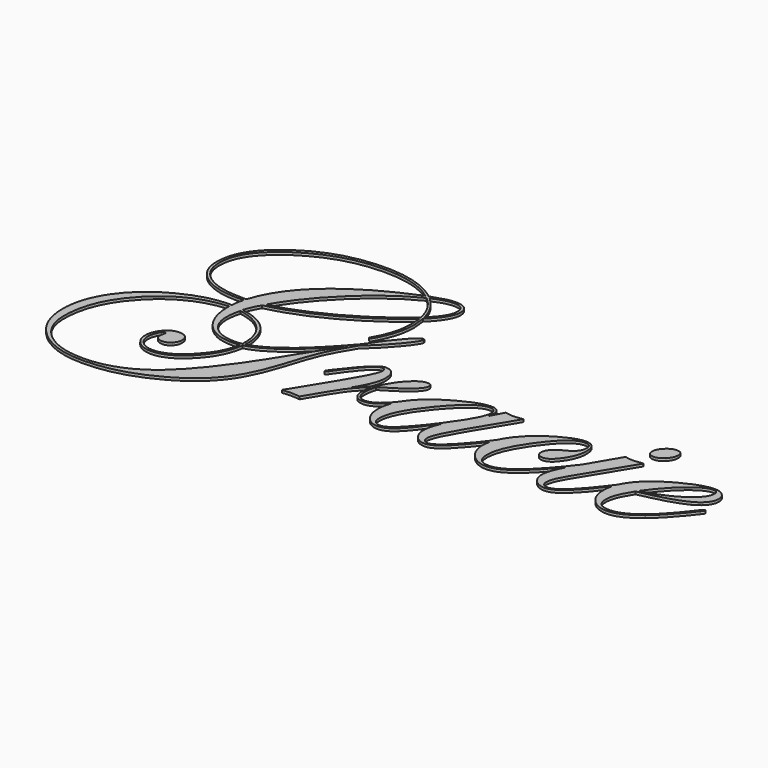
from build123d import *

# Parameters (mm, degrees)
F1_DEPTH = 1.5


# Not quite as in the source:
# - ends of sketch curves that miss each other by under 0.0002 mm in the source are joined


with BuildPart() as f1:
    # F0 (on Top) → F1 (new body)
    with BuildSketch(Plane.XY):
        with BuildLine():
            add(Edge.make_bspline(
                [(-28.4636718, 33.839658), (-28.4636718, 32.4505066), (-30.630749, 29.1998908), (-34.964878, 24.087836)],
                knots=[0, 0, 0, 0, 1, 1, 1, 1], degree=3))
            add(Edge.make_bspline(
                [(-29.1304218, 34.3397078), (-28.7970468, 34.3397078), (-28.5747714, 34.173033), (-28.4636718, 33.839658)],
                knots=[0, 0, 0, 0, 1, 1, 1, 1], degree=3))
            add(Edge.make_bspline(
                [(-36.8818668, 27.8385016), (-33.1033882, 32.172656), (-30.5195732, 34.3397078), (-29.1304218, 34.3397078)],
                knots=[0, 0, 0, 0, 1, 1, 1, 1], degree=3))
            add(Edge.make_bspline(
                [(-47.967265, 12.8356868), (-44.3554866, 18.5034174), (-40.6603454, 23.5043472), (-36.8818668, 27.8385016)],
                knots=[0, 0, 0, 0, 1, 1, 1, 1], degree=3))
            add(Edge.make_bspline(
                [(-88.7248924, -20.0871328), (-77.6672818, -17.0865546), (-64.081406, -6.1122814), (-47.967265, 12.8356868)],
                knots=[0, 0, 0, 0, 1, 1, 1, 1], degree=3))
            Line((-88.7248924, -20.0871328), (-88.7248924, -18.4201562))
            add(Edge.make_bspline(
                [(-110.729014, 5.5009796), (-96.0595996, 3.0005274), (-88.7248924, -4.973193), (-88.7248924, -18.4201562)],
                knots=[0, 0, 0, 0, 1, 1, 1, 1], degree=3))
            add(Edge.make_bspline(
                [(-106.6449226, 14.5026634), (-108.4230242, 11.6132356), (-109.784388, 8.6126828), (-110.729014, 5.5009796)],
                knots=[0, 0, 0, 0, 1, 1, 1, 1], degree=3))
            add(Edge.make_bspline(
                [(-74.055478, 27.0883634), (-85.4465144, 21.0316826), (-96.3096372, 16.8364408), (-106.6449226, 14.5026634)],
                knots=[0, 0, 0, 0, 1, 1, 1, 1], degree=3))
            add(Edge.make_bspline(
                [(-42.9663352, 48.5090216), (-52.2458442, 40.3408388), (-62.6088918, 33.2006194), (-74.055478, 27.0883634)],
                knots=[0, 0, 0, 0, 1, 1, 1, 1], degree=3))
            add(Edge.make_bspline(
                [(-42.6329348, 42.1745156), (-42.6329348, 44.4527178), (-42.7440852, 46.5642198), (-42.9663352, 48.5090216)],
                knots=[0, 0, 0, 0, 1, 1, 1, 1], degree=3))
            add(Edge.make_bspline(
                [(-48.800766, 20.8371948), (-44.688887, 27.6162262), (-42.6329348, 34.7286834), (-42.6329348, 42.1745156)],
                knots=[0, 0, 0, 0, 1, 1, 1, 1], degree=3))
            add(Edge.make_bspline(
                [(-49.1341664, 20.0036938), (-49.0786166, 20.281519), (-48.9674662, 20.5593442), (-48.800766, 20.8371948)],
                knots=[0, 0, 0, 0, 1, 1, 1, 1], degree=3))
            add(Edge.make_bspline(
                [(-48.6340912, 19.503644), (-48.9119164, 19.503644), (-49.0786166, 19.6703188), (-49.1341664, 20.0036938)],
                knots=[0, 0, 0, 0, 1, 1, 1, 1], degree=3))
            add(Edge.make_bspline(
                [(-46.3836766, 22.5875596), (-47.4394276, 20.5316074), (-48.1895658, 19.503644), (-48.6340912, 19.503644)],
                knots=[0, 0, 0, 0, 1, 1, 1, 1], degree=3))
            add(Edge.make_bspline(
                [(-41.1326838, 41.8411406), (-41.1326838, 35.840035), (-42.8830232, 29.4221662), (-46.3836766, 22.5875596)],
                knots=[0, 0, 0, 0, 1, 1, 1, 1], degree=3))
            add(Edge.make_bspline(
                [(-41.7994846, 49.5092482), (-41.3549592, 46.4531202), (-41.1326838, 43.8970928), (-41.1326838, 41.8411406)],
                knots=[0, 0, 0, 0, 1, 1, 1, 1], degree=3))
            add(Edge.make_bspline(
                [(-32.381063, 64.845438), (-32.381063, 60.733559), (-35.5205538, 55.6215042), (-41.7994846, 49.5092482)],
                knots=[0, 0, 0, 0, 1, 1, 1, 1], degree=3))
            add(Edge.make_bspline(
                [(-40.4659084, 71.5133698), (-35.076003, 71.5133698), (-32.381063, 69.2907174), (-32.381063, 64.845438)],
                knots=[0, 0, 0, 0, 1, 1, 1, 1], degree=3))
            add(Edge.make_bspline(
                [(-53.3850088, 68.262754), (-47.550578, 70.4298312), (-43.2442112, 71.5133698), (-40.4659084, 71.5133698)],
                knots=[0, 0, 0, 0, 1, 1, 1, 1], degree=3))
            add(Edge.make_bspline(
                [(-85.8077278, 78.1812762), (-72.5830146, 78.1812762), (-61.7754416, 74.8751106), (-53.3850088, 68.262754)],
                knots=[0, 0, 0, 0, 1, 1, 1, 1], degree=3))
            add(Edge.make_bspline(
                [(-130.0660086, 65.0121382), (-117.230271, 73.791572), (-102.4774938, 78.1812762), (-85.8077278, 78.1812762)],
                knots=[0, 0, 0, 0, 1, 1, 1, 1], degree=3))
            add(Edge.make_bspline(
                [(-149.3195896, 34.8398338), (-149.3195896, 46.175295), (-142.9017208, 56.2327298), (-130.0660086, 65.0121382)],
                knots=[0, 0, 0, 0, 1, 1, 1, 1], degree=3))
            add(Edge.make_bspline(
                [(-141.4014444, 19.0868808), (-146.6802248, 23.032085), (-149.3195896, 28.2830524), (-149.3195896, 34.8398338)],
                knots=[0, 0, 0, 0, 1, 1, 1, 1], degree=3))
            add(Edge.make_bspline(
                [(-119.9807862, 13.1691126), (-128.9268948, 13.1691126), (-136.0671142, 15.141702), (-141.4014444, 19.0868808)],
                knots=[0, 0, 0, 0, 1, 1, 1, 1], degree=3))
            add(Edge.make_bspline(
                [(-116.39677, 13.3357874), (-117.3969712, 13.2246878), (-118.5916348, 13.1691126), (-119.9807862, 13.1691126)],
                knots=[0, 0, 0, 0, 1, 1, 1, 1], degree=3))
            add(Edge.make_bspline(
                [(-117.563646, 6.0010802), (-117.5636714, 7.3902316), (-117.1746958, 9.835134), (-116.39677, 13.3357874)],
                knots=[0, 0, 0, 0, 1, 1, 1, 1], degree=3))
            add(Edge.make_bspline(
                [(-119.3139854, 6.1678312), (-118.6471846, 6.1678312), (-118.0637466, 6.1122306), (-117.563646, 6.0010802)],
                knots=[0, 0, 0, 0, 1, 1, 1, 1], degree=3))
            add(Edge.make_bspline(
                [(-145.068798, -1.0002012), (-135.789289, 3.7784786), (-127.204343, 6.1678312), (-119.3139854, 6.1678312)],
                knots=[0, 0, 0, 0, 1, 1, 1, 1], degree=3))
            add(Edge.make_bspline(
                [(-166.9062194, -19.8370444), (-161.5718892, -12.0578118), (-154.2927572, -5.7788556), (-145.068798, -1.0002012)],
                knots=[0, 0, 0, 0, 1, 1, 1, 1], degree=3))
            add(Edge.make_bspline(
                [(-174.907702, -44.3416436), (-174.907702, -35.72891), (-172.2405496, -27.5607018), (-166.9062194, -19.8370444)],
                knots=[0, 0, 0, 0, 1, 1, 1, 1], degree=3))
            add(Edge.make_bspline(
                [(-164.3224044, -68.8462428), (-171.3792864, -62.622811), (-174.907702, -54.4546282), (-174.907702, -44.3416436)],
                knots=[0, 0, 0, 0, 1, 1, 1, 1], degree=3))
            add(Edge.make_bspline(
                [(-136.5672148, -78.1813016), (-148.013801, -78.1813016), (-157.2655224, -75.0696238), (-164.3224044, -68.8462428)],
                knots=[0, 0, 0, 0, 1, 1, 1, 1], degree=3))
            add(Edge.make_bspline(
                [(-96.9764634, -67.4293038), (-109.8677762, -74.5973108), (-123.0646764, -78.1813016), (-136.5672148, -78.1813016)],
                knots=[0, 0, 0, 0, 1, 1, 1, 1], degree=3))
            add(Edge.make_bspline(
                [(-76.0559058, -50.3427746), (-81.0012604, -56.7328304), (-87.974805, -62.4283232), (-96.9764634, -67.4293038)],
                knots=[0, 0, 0, 0, 1, 1, 1, 1], degree=3))
            add(Edge.make_bspline(
                [(-63.4702058, -24.4212364), (-66.8597342, -35.3121722), (-71.054976, -43.9526934), (-76.0559058, -50.3427746)],
                knots=[0, 0, 0, 0, 1, 1, 1, 1], degree=3))
            add(Edge.make_bspline(
                [(-56.6355992, -4.834255), (-58.469276, -8.9461086), (-60.7474782, -15.4751278), (-63.4702058, -24.4212364)],
                knots=[0, 0, 0, 0, 1, 1, 1, 1], degree=3))
            add(Edge.make_bspline(
                [(-47.9673158, 10.918698), (-51.9124946, 4.584192), (-54.8019224, -0.6668008), (-56.6355992, -4.834255)],
                knots=[0, 0, 0, 0, 1, 1, 1, 1], degree=3))
            add(Edge.make_bspline(
                [(-34.964878, 24.087836), (-39.2434572, 19.031331), (-43.5776116, 14.6416268), (-47.9673158, 10.918698)],
                knots=[0, 0, 0, 0, 1, 1, 1, 1], degree=3))
        make_face()
        with BuildLine():
            add(Edge.make_bspline(
                [(-50.8845312, 7.5014074), (-65.8317708, -9.1128088), (-78.556358, -18.8368432), (-89.0583436, -21.6707212)],
                knots=[0, 0, 0, 0, 1, 1, 1, 1], degree=3))
            add(Edge.make_bspline(
                [(-64.6371072, -13.1691634), (-60.3029528, -5.8344562), (-55.7187608, 1.0557256), (-50.8845312, 7.5014074)],
                knots=[0, 0, 0, 0, 1, 1, 1, 1], degree=3))
            add(Edge.make_bspline(
                [(-101.9774186, -62.5117368), (-91.253183, -53.2322278), (-78.806421, -36.7847118), (-64.6371072, -13.1691634)],
                knots=[0, 0, 0, 0, 1, 1, 1, 1], degree=3))
            add(Edge.make_bspline(
                [(-137.7340908, -76.4309876), (-124.620528, -76.4309876), (-112.7016288, -71.7912458), (-101.9774186, -62.5117368)],
                knots=[0, 0, 0, 0, 1, 1, 1, 1], degree=3))
            add(Edge.make_bspline(
                [(-161.2384888, -68.9296056), (-155.2373578, -73.9305354), (-147.4025754, -76.4309876), (-137.7340908, -76.4309876)],
                knots=[0, 0, 0, 0, 1, 1, 1, 1], degree=3))
            add(Edge.make_bspline(
                [(-170.1568352, -49.3425988), (-170.1568352, -57.399682), (-167.1840446, -63.9286758), (-161.2384888, -68.9296056)],
                knots=[0, 0, 0, 0, 1, 1, 1, 1], degree=3))
            add(Edge.make_bspline(
                [(-154.4872196, -13.0858006), (-164.93363, -23.8100362), (-170.1568352, -35.8956356), (-170.1568352, -49.3425988)],
                knots=[0, 0, 0, 0, 1, 1, 1, 1], degree=3))
            add(Edge.make_bspline(
                [(-117.7303462, 4.4174664), (-131.7329852, 3.5284156), (-143.9852594, -2.3060152), (-154.4872196, -13.0858006)],
                knots=[0, 0, 0, 0, 1, 1, 1, 1], degree=3))
            add(Edge.make_bspline(
                [(-111.5625404, -15.1695404), (-115.6744194, -10.3352854), (-117.7303462, -3.8062916), (-117.7303462, 4.4174664)],
                knots=[0, 0, 0, 0, 1, 1, 1, 1], degree=3))
            add(Edge.make_bspline(
                [(-94.7260488, -22.3375474), (-101.838506, -22.3375474), (-107.4506614, -19.9481948), (-111.5625404, -15.1695404)],
                knots=[0, 0, 0, 0, 1, 1, 1, 1], degree=3))
            add(Edge.make_bspline(
                [(-90.4752572, -22.004147), (-91.6977084, -22.226397), (-93.1146474, -22.3375474), (-94.7260488, -22.3375474)],
                knots=[0, 0, 0, 0, 1, 1, 1, 1], degree=3))
            add(Edge.make_bspline(
                [(-100.643817, -41.2577534), (-94.6427114, -35.0899222), (-91.253183, -28.6720534), (-90.4752572, -22.004147)],
                knots=[0, 0, 0, 0, 1, 1, 1, 1], degree=3))
            add(Edge.make_bspline(
                [(-118.0637466, -50.5094748), (-112.396016, -50.5094748), (-106.5893728, -47.4255592), (-100.643817, -41.2577534)],
                knots=[0, 0, 0, 0, 1, 1, 1, 1], degree=3))
            add(Edge.make_bspline(
                [(-125.1484162, -47.9256852), (-123.2591642, -49.6482116), (-120.8976246, -50.5094748), (-118.0637466, -50.5094748)],
                knots=[0, 0, 0, 0, 1, 1, 1, 1], degree=3))
            add(Edge.make_bspline(
                [(-127.9822688, -41.4244028), (-127.9822688, -44.0360054), (-127.0376428, -46.203108), (-125.1484162, -47.9256852)],
                knots=[0, 0, 0, 0, 1, 1, 1, 1], degree=3))
            add(Edge.make_bspline(
                [(-126.73203, -36.3401356), (-127.565531, -38.118288), (-127.9822688, -39.8130268), (-127.9822688, -41.4244028)],
                knots=[0, 0, 0, 0, 1, 1, 1, 1], degree=3))
            add(Edge.make_bspline(
                [(-124.2315778, -33.5896458), (-125.0650534, -33.5896458), (-125.8985544, -34.5064842), (-126.73203, -36.3401356)],
                knots=[0, 0, 0, 0, 1, 1, 1, 1], degree=3))
            add(Edge.make_bspline(
                [(-123.7315026, -34.0896956), (-123.7315026, -33.7563206), (-123.8982028, -33.5896458), (-124.2315778, -33.5896458)],
                knots=[0, 0, 0, 0, 1, 1, 1, 1], degree=3))
            add(Edge.make_bspline(
                [(-123.8981774, -35.339909), (-123.7870524, -34.8953836), (-123.7315026, -34.4786458), (-123.7315026, -34.0896956)],
                knots=[0, 0, 0, 0, 1, 1, 1, 1], degree=3))
            add(Edge.make_bspline(
                [(-124.2315778, -37.1735858), (-124.2315778, -36.7846864), (-124.1204528, -36.1734862), (-123.8981774, -35.339909)],
                knots=[0, 0, 0, 0, 1, 1, 1, 1], degree=3))
            add(Edge.make_bspline(
                [(-119.814086, -41.090977), (-122.7590636, -41.090977), (-124.2315778, -39.7851884), (-124.2315778, -37.1735858)],
                knots=[0, 0, 0, 0, 1, 1, 1, 1], degree=3))
            add(Edge.make_bspline(
                [(-115.5632944, -39.1739882), (-116.8412954, -40.4519892), (-118.2582344, -41.090977), (-119.814086, -41.090977)],
                knots=[0, 0, 0, 0, 1, 1, 1, 1], degree=3))
            add(Edge.make_bspline(
                [(-113.6462548, -34.8398592), (-113.6462548, -36.451286), (-114.285268, -37.8959872), (-115.5632944, -39.1739882)],
                knots=[0, 0, 0, 0, 1, 1, 1, 1], degree=3))
            add(Edge.make_bspline(
                [(-119.4806856, -29.505529), (-115.5910566, -29.505529), (-113.6462548, -31.2836306), (-113.6462548, -34.8398592)],
                knots=[0, 0, 0, 0, 1, 1, 1, 1], degree=3))
            add(Edge.make_bspline(
                [(-126.4819924, -33.1728572), (-124.3704904, -30.7279802), (-122.036713, -29.505529), (-119.4806856, -29.505529)],
                knots=[0, 0, 0, 0, 1, 1, 1, 1], degree=3))
            add(Edge.make_bspline(
                [(-129.565908, -41.4243774), (-129.565908, -38.3683002), (-128.5379446, -35.617785), (-126.4819924, -33.1728572)],
                knots=[0, 0, 0, 0, 1, 1, 1, 1], degree=3))
            add(Edge.make_bspline(
                [(-126.3152922, -48.8424474), (-128.4823694, -46.8420958), (-129.565908, -44.3694058), (-129.565908, -41.4243774)],
                knots=[0, 0, 0, 0, 1, 1, 1, 1], degree=3))
            add(Edge.make_bspline(
                [(-118.0637466, -51.843051), (-121.34215, -51.843051), (-124.0926652, -50.8428498), (-126.3152922, -48.8424474)],
                knots=[0, 0, 0, 0, 1, 1, 1, 1], degree=3))
            add(Edge.make_bspline(
                [(-99.8103414, -42.507916), (-105.8114724, -48.7313478), (-111.8959408, -51.843051), (-118.0637466, -51.843051)],
                knots=[0, 0, 0, 0, 1, 1, 1, 1], degree=3))
            add(Edge.make_bspline(
                [(-89.0583436, -21.6707212), (-90.1696444, -29.2832536), (-93.7536606, -36.2289852), (-99.8103414, -42.507916)],
                knots=[0, 0, 0, 0, 1, 1, 1, 1], degree=3))
        make_face(mode=Mode.SUBTRACT)
        with BuildLine():
            add(Edge.make_bspline(
                [(-90.1418568, -20.5038452), (-89.7528812, -13.8914886), (-91.3920702, -8.4460334), (-95.0594492, -4.1674542)],
                knots=[0, 0, 0, 0, 1, 1, 1, 1], degree=3))
            add(Edge.make_bspline(
                [(-94.7260488, -20.8372202), (-93.1146474, -20.8372202), (-91.5865834, -20.7260952), (-90.1418568, -20.5038452)],
                knots=[0, 0, 0, 0, 1, 1, 1, 1], degree=3))
            add(Edge.make_bspline(
                [(-107.3950862, -16.336391), (-104.172258, -19.3369438), (-99.949254, -20.8372202), (-94.7260488, -20.8372202)],
                knots=[0, 0, 0, 0, 1, 1, 1, 1], degree=3))
            add(Edge.make_bspline(
                [(-112.1459784, -4.4174918), (-112.1459784, -9.3628718), (-110.5623392, -13.3358382), (-107.3950862, -16.336391)],
                knots=[0, 0, 0, 0, 1, 1, 1, 1], degree=3))
            add(Edge.make_bspline(
                [(-110.8957396, 4.0840914), (-111.7292406, 1.2502388), (-112.1459784, -1.5836392), (-112.1459784, -4.4174918)],
                knots=[0, 0, 0, 0, 1, 1, 1, 1], degree=3))
            add(Edge.make_bspline(
                [(-95.0594492, -4.1674542), (-98.7268028, 0.1667002), (-104.0055578, 2.9172154), (-110.8957396, 4.0840914)],
                knots=[0, 0, 0, 0, 1, 1, 1, 1], degree=3))
        make_face(mode=Mode.SUBTRACT)
        with BuildLine():
            add(Edge.make_bspline(
                [(-54.9686226, 67.7626788), (-62.358905, 73.5970842), (-72.5274648, 76.5142996), (-85.4743274, 76.5142996)],
                knots=[0, 0, 0, 0, 1, 1, 1, 1], degree=3))
            add(Edge.make_bspline(
                [(-115.8966694, 14.6694144), (-109.3954632, 35.95116), (-89.0861058, 53.6489148), (-54.9686226, 67.7626788)],
                knots=[0, 0, 0, 0, 1, 1, 1, 1], degree=3))
            Line((-115.8966694, 14.6694144), (-118.8138848, 14.6694144))
            add(Edge.make_bspline(
                [(-140.1512056, 20.0037446), (-135.0391508, 16.447516), (-127.926719, 14.6694144), (-118.8138848, 14.6694144)],
                knots=[0, 0, 0, 0, 1, 1, 1, 1], degree=3))
            add(Edge.make_bspline(
                [(-147.8193132, 35.006534), (-147.8193132, 28.6164528), (-145.2632858, 23.615523), (-140.1512056, 20.0037446)],
                knots=[0, 0, 0, 0, 1, 1, 1, 1], degree=3))
            add(Edge.make_bspline(
                [(-128.399032, 63.5118618), (-141.3458946, 54.8991536), (-147.8193132, 45.3973692), (-147.8193132, 35.006534)],
                knots=[0, 0, 0, 0, 1, 1, 1, 1], degree=3))
            add(Edge.make_bspline(
                [(-85.4743274, 76.5142996), (-101.0883678, 76.5142996), (-115.3965942, 72.1801706), (-128.399032, 63.5118618)],
                knots=[0, 0, 0, 0, 1, 1, 1, 1], degree=3))
        make_face(mode=Mode.SUBTRACT)
        with BuildLine():
            add(Edge.make_bspline(
                [(-43.2997864, 50.0093488), (-44.7444876, 56.6217054), (-48.0506532, 62.0949482), (-53.2183086, 66.4290772)],
                knots=[0, 0, 0, 0, 1, 1, 1, 1], degree=3))
            add(Edge.make_bspline(
                [(-73.972166, 28.7553654), (-62.581155, 34.9231966), (-52.35702, 42.0078408), (-43.2997864, 50.0093488)],
                knots=[0, 0, 0, 0, 1, 1, 1, 1], degree=3))
            add(Edge.make_bspline(
                [(-105.8114724, 16.0863534), (-95.9207378, 18.4201054), (-85.3076272, 22.6431094), (-73.972166, 28.7553654)],
                knots=[0, 0, 0, 0, 1, 1, 1, 1], degree=3))
            add(Edge.make_bspline(
                [(-82.8905124, 44.8417188), (-92.7256718, 35.4510594), (-100.3659918, 25.8659376), (-105.8114724, 16.0863534)],
                knots=[0, 0, 0, 0, 1, 1, 1, 1], degree=3))
            add(Edge.make_bspline(
                [(-53.2183086, 66.4290772), (-63.164593, 61.4837226), (-73.0553276, 54.287928), (-82.8905124, 44.8417188)],
                knots=[0, 0, 0, 0, 1, 1, 1, 1], degree=3))
        make_face(mode=Mode.SUBTRACT)
        with BuildLine():
            add(Edge.make_bspline(
                [(-33.9647022, 64.6787632), (-33.9647022, 68.3461168), (-36.0762042, 70.1797936), (-40.2992082, 70.1797936)],
                knots=[0, 0, 0, 0, 1, 1, 1, 1], degree=3))
            add(Edge.make_bspline(
                [(-42.132885, 51.0928874), (-36.6874298, 56.3716424), (-33.9647022, 60.9002846), (-33.9647022, 64.6787632)],
                knots=[0, 0, 0, 0, 1, 1, 1, 1], degree=3))
            add(Edge.make_bspline(
                [(-51.884707, 66.9291778), (-47.1060526, 62.8172988), (-43.8554368, 57.5385438), (-42.132885, 51.0928874)],
                knots=[0, 0, 0, 0, 1, 1, 1, 1], degree=3))
            add(Edge.make_bspline(
                [(-40.2992082, 70.1797936), (-43.5220364, 70.1797936), (-47.3838778, 69.096255), (-51.884707, 66.9291778)],
                knots=[0, 0, 0, 0, 1, 1, 1, 1], degree=3))
        make_face(mode=Mode.SUBTRACT)
    extrude(amount=F1_DEPTH)


with BuildPart() as f1b:
    # F0 (on Top) → F1, piece 2 (new body)
    with BuildSketch(Plane.XY):
        with BuildLine():
            add(Edge.make_bspline(
                [(3.8757098, -16.753078), (4.2090848, -16.753078), (4.375785, -16.9197782), (4.375785, -17.2531532)],
                knots=[0, 0, 0, 0, 1, 1, 1, 1], degree=3))
            add(Edge.make_bspline(
                [(4.375785, -17.2531532), (4.3758104, -17.6977548), (2.7088338, -19.7259194), (-0.6251448, -23.3376978)],
                knots=[0, 0, 0, 0, 1, 1, 1, 1], degree=3))
            add(Edge.make_bspline(
                [(-0.6251448, -23.3376978), (-0.7840491374, -23.5133298152), (-0.9425994498, -23.6856574299), (-1.100795736, -23.8546806469)],
                knots=[0, 0, 0, 0, 0.0376282706, 0.0376282706, 0.0376282706, 0.0376282706], degree=3))
            add(Edge.make_bspline(
                [(-2.6254964, -31.9226438), (-2.6254964, -29.150805094), (-2.1172629938, -26.4614841914), (-1.100795736, -23.8546806469)],
                knots=[0, 0, 0, 0, 0.2598113167, 0.2598113167, 0.2598113167, 0.2598113167], degree=3))
            add(Edge.make_bspline(
                [(0.3750564, -41.507791), (-1.6253206, -38.9517382), (-2.6254964, -35.7566976), (-2.6254964, -31.9226438)],
                knots=[0, 0, 0, 0, 1, 1, 1, 1], degree=3))
            add(Edge.make_bspline(
                [(7.793101, -45.2584566), (4.848098, -45.2584566), (2.3754334, -44.0082178), (0.3750564, -41.507791)],
                knots=[0, 0, 0, 0, 1, 1, 1, 1], degree=3))
            add(Edge.make_bspline(
                [(16.378047, -41.1743906), (13.433044, -43.8970928), (10.5714038, -45.2584566), (7.793101, -45.2584566)],
                knots=[0, 0, 0, 0, 1, 1, 1, 1], degree=3))
            add(Edge.make_bspline(
                [(29.1304218, -25.4214122), (23.5738416, -33.2006448), (19.3230246, -38.4516376), (16.378047, -41.1743906)],
                knots=[0, 0, 0, 0, 1, 1, 1, 1], degree=3))
            add(Edge.make_bspline(
                [(26.4632694, -35.1732596), (26.4632694, -32.1726814), (27.3523202, -28.9220656), (29.1304218, -25.4214122)],
                knots=[0, 0, 0, 0, 1, 1, 1, 1], degree=3))
            add(Edge.make_bspline(
                [(28.8803842, -42.4245786), (27.2689574, -40.4797768), (26.4632694, -38.062662), (26.4632694, -35.1732596)],
                knots=[0, 0, 0, 0, 1, 1, 1, 1], degree=3))
            add(Edge.make_bspline(
                [(35.1315528, -45.2584566), (32.5755, -45.2584566), (30.4917856, -44.3138306), (28.8803842, -42.4245786)],
                knots=[0, 0, 0, 0, 1, 1, 1, 1], degree=3))
            add(Edge.make_bspline(
                [(50.6344428, -33.4229202), (44.0776614, -41.3132778), (38.9100314, -45.2584566), (35.1315528, -45.2584566)],
                knots=[0, 0, 0, 0, 1, 1, 1, 1], degree=3))
            add(Edge.make_bspline(
                [(57.0452664146, -25.6560193697), (55.3034828285, -27.8335905942), (53.1665418811, -30.4225577951), (50.6344428, -33.4229202)],
                knots=[0.6878819637, 0.6878819637, 0.6878819637, 0.6878819637, 1, 1, 1, 1], degree=3))
            add(Edge.make_bspline(
                [(57.0452664146, -25.6560193697), (57.3568975946, -24.4213866988), (57.7948929281, -23.1756034866), (58.3592519758, -21.9186706118)],
                knots=[0.318899631, 0.318899631, 0.318899631, 0.318899631, 0.5775230996, 0.5775230996, 0.5775230996, 0.5775230996], degree=3))
            add(Edge.make_bspline(
                [(46.4669886, -36.4234476), (50.3777652225, -32.3349194844), (54.341848683, -27.499998153), (58.3592519758, -21.9186706118)],
                knots=[0, 0, 0, 0, 0.7997817464, 0.7997817464, 0.7997817464, 0.7997817464], degree=3))
            add(Edge.make_bspline(
                [(35.7983282, -44.0082432), (38.0209806, -44.0082432), (41.5771838, -41.479978), (46.4669886, -36.4234476)],
                knots=[0, 0, 0, 0, 1, 1, 1, 1], degree=3))
            add(Edge.make_bspline(
                [(32.5477378, -40.090852), (32.5477378, -42.7024546), (33.631251, -44.0082432), (35.7983282, -44.0082432)],
                knots=[0, 0, 0, 0, 1, 1, 1, 1], degree=3))
            add(Edge.make_bspline(
                [(40.21582, -23.1709976), (35.1037652, -31.728156), (32.5477378, -37.368099), (32.5477378, -40.090852)],
                knots=[0, 0, 0, 0, 1, 1, 1, 1], degree=3))
            Line((40.21582, -23.1709976), (54.9685718, 1.2502388))
            add(Edge.make_bspline(
                [(49.1341664, 0.6667754), (50.6344428, 0.6667754), (52.5792446, 0.8612632), (54.9685718, 1.2502388)],
                knots=[0, 0, 0, 0, 1, 1, 1, 1], degree=3))
            add(Edge.make_bspline(
                [(44.7166746, 1.2502388), (46.3836512, 0.8612632), (47.85614, 0.6667754), (49.1341664, 0.6667754)],
                knots=[0, 0, 0, 0, 1, 1, 1, 1], degree=3))
            Line((44.7166746, 1.2502388), (40.465883, -6.8346066))
            add(Edge.make_bspline(
                [(41.1326584, -3.0839156), (41.1326584, -4.0285416), (40.9104084, -5.278755), (40.465883, -6.8346066)],
                knots=[0, 0, 0, 0, 1, 1, 1, 1], degree=3))
            add(Edge.make_bspline(
                [(35.9650284, 1.9170142), (39.410132, 1.9170142), (41.1326584, 0.2500376), (41.1326584, -3.0839156)],
                knots=[0, 0, 0, 0, 1, 1, 1, 1], degree=3))
            add(Edge.make_bspline(
                [(19.9620378, -3.5839908), (26.5743944, 0.0833374), (31.9087246, 1.9170142), (35.9650284, 1.9170142)],
                knots=[0, 0, 0, 0, 1, 1, 1, 1], degree=3))
            add(Edge.make_bspline(
                [(1.0616458883, -19.5900044112), (4.6875343472, -13.8204774935), (10.9876631922, -8.4851414153), (19.9620378, -3.5839908)],
                knots=[0.4040272735, 0.4040272735, 0.4040272735, 0.4040272735, 1, 1, 1, 1], degree=3))
            add(Edge.make_bspline(
                [(1.0616458883, -19.5900044112), (1.3042071167, -19.263775449), (1.5476569539, -18.929358911), (1.7919954, -18.5867548)],
                knots=[0.9522037142, 0.9522037142, 0.9522037142, 0.9522037142, 1, 1, 1, 1], degree=3))
            add(Edge.make_bspline(
                [(1.7919954, -18.5867548), (2.9032962, -17.3643036), (3.5978846, -16.753078), (3.8757098, -16.753078)],
                knots=[0, 0, 0, 0, 1, 1, 1, 1], degree=3))
        make_face()
        with BuildLine():
            add(Edge.make_bspline(
                [(39.882445, -3.417316), (39.882445, -0.6945884), (38.6322062, 0.6668008), (36.1317286, 0.6668008)],
                knots=[0, 0, 0, 0, 1, 1, 1, 1], degree=3))
            add(Edge.make_bspline(
                [(28.2969462, -24.921337), (36.0206036, -14.4749266), (39.882445, -7.3069196), (39.882445, -3.417316)],
                knots=[0, 0, 0, 0, 1, 1, 1, 1], degree=3))
            add(Edge.make_bspline(
                [(8.376539, -44.0082432), (12.2105928, -44.0082432), (18.850737, -37.6459496), (28.2969462, -24.921337)],
                knots=[0, 0, 0, 0, 1, 1, 1, 1], degree=3))
            add(Edge.make_bspline(
                [(3.5423094, -38.5905248), (3.5423094, -42.2023286), (5.1537108, -44.0082432), (8.376539, -44.0082432)],
                knots=[0, 0, 0, 0, 1, 1, 1, 1], degree=3))
            add(Edge.make_bspline(
                [(15.9612838, -14.336014), (7.681976, -24.337899), (3.5423094, -32.422719), (3.5423094, -38.5905248)],
                knots=[0, 0, 0, 0, 1, 1, 1, 1], degree=3))
            add(Edge.make_bspline(
                [(36.1317286, 0.6668008), (31.0196738, 0.6668008), (24.2961922, -4.3341544), (15.9612838, -14.336014)],
                knots=[0, 0, 0, 0, 1, 1, 1, 1], degree=3))
        make_face(mode=Mode.SUBTRACT)
        with BuildLine():
            add(Edge.make_bspline(
                [(4.3758104, -17.2532294), (4.3758104, -17.6977548), (2.7088338, -19.7259194), (-0.6251448, -23.3376978)],
                knots=[0, 0, 0, 0, 1, 1, 1, 1], degree=3))
            add(Edge.make_bspline(
                [(3.8757098, -16.753078), (4.2090848, -16.753078), (4.375785, -16.9197782), (4.3758104, -17.2532294)],
                knots=[0, 0, 0, 0, 1, 1, 1, 1], degree=3))
            add(Edge.make_bspline(
                [(1.7919954, -18.5867548), (2.9032962, -17.3643036), (3.5978846, -16.753078), (3.8757098, -16.753078)],
                knots=[0, 0, 0, 0, 1, 1, 1, 1], degree=3))
            add(Edge.make_bspline(
                [(1.0616458883, -19.5900044112), (1.3042071167, -19.263775449), (1.5476569539, -18.929358911), (1.7919954, -18.5867548)],
                knots=[0.9522037142, 0.9522037142, 0.9522037142, 0.9522037142, 1, 1, 1, 1], degree=3))
            add(Edge.make_bspline(
                [(-1.100795736, -23.8546806469), (-0.5365755167, -22.4076972282), (0.1842383327, -20.9861385083), (1.0616458883, -19.5900044112)],
                knots=[0.2598113167, 0.2598113167, 0.2598113167, 0.2598113167, 0.4040272735, 0.4040272735, 0.4040272735, 0.4040272735], degree=3))
            add(Edge.make_bspline(
                [(-0.6251448, -23.3376978), (-0.7840491374, -23.5133298152), (-0.9425994498, -23.6856574299), (-1.100795736, -23.8546806469)],
                knots=[0, 0, 0, 0, 0.0376282706, 0.0376282706, 0.0376282706, 0.0376282706], degree=3))
        make_face()
        with BuildLine():
            add(Edge.make_bspline(
                [(-1.100795736, -23.8546806469), (-5.1467864489, -28.1775783751), (-8.9612016167, -30.3390046), (-12.5440186, -30.3390046)],
                knots=[0.0376282706, 0.0376282706, 0.0376282706, 0.0376282706, 1, 1, 1, 1], degree=3))
            add(Edge.make_bspline(
                [(-1.100795736, -23.8546806469), (-0.5365755167, -22.4076972282), (0.1842383327, -20.9861385083), (1.0616458883, -19.5900044112)],
                knots=[0.2598113167, 0.2598113167, 0.2598113167, 0.2598113167, 0.4040272735, 0.4040272735, 0.4040272735, 0.4040272735], degree=3))
            add(Edge.make_bspline(
                [(-12.3773184, -29.338778), (-8.2503446682, -29.338778), (-3.7706899055, -26.089179494), (1.0616458883, -19.5900044112)],
                knots=[0, 0, 0, 0, 0.9522037142, 0.9522037142, 0.9522037142, 0.9522037142], degree=3))
            add(Edge.make_bspline(
                [(-17.6283112, -22.3374712), (-17.6283112, -27.0050006), (-15.8779972, -29.338778), (-12.3773184, -29.338778)],
                knots=[0, 0, 0, 0, 1, 1, 1, 1], degree=3))
            add(Edge.make_bspline(
                [(-16.4614352, -16.0029398), (-17.239361, -18.5589672), (-17.6283112, -20.6704946), (-17.6283112, -22.3374712)],
                knots=[0, 0, 0, 0, 1, 1, 1, 1], degree=3))
            Line((-16.4614352, -16.0029398), (-15.461234, -15.1694642))
            add(Edge.make_bspline(
                [(-9.9602036, -11.7521482), (-11.1826548, -12.530074), (-13.0163316, -13.6691878), (-15.461234, -15.1694642)],
                knots=[0, 0, 0, 0, 1, 1, 1, 1], degree=3))
            add(Edge.make_bspline(
                [(1.6252952, -0.3333496), (1.6252952, -3.000502), (-2.2365462, -6.8067936), (-9.9602036, -11.7521482)],
                knots=[0, 0, 0, 0, 1, 1, 1, 1], degree=3))
            add(Edge.make_bspline(
                [(-0.9585198, 1.917065), (0.7640066, 1.917065), (1.6252952, 1.1669268), (1.6252952, -0.3333496)],
                knots=[0, 0, 0, 0, 1, 1, 1, 1], degree=3))
            add(Edge.make_bspline(
                [(-9.4601284, -3.0838648), (-6.29285, 0.2500884), (-3.4589974, 1.917065), (-0.9585198, 1.917065)],
                knots=[0, 0, 0, 0, 1, 1, 1, 1], degree=3))
            add(Edge.make_bspline(
                [(-17.2949108, -15.5028392), (-15.1834088, -10.5574846), (-12.5718062, -6.417818), (-9.4601284, -3.0838648)],
                knots=[0, 0, 0, 0, 1, 1, 1, 1], degree=3))
            add(Edge.make_bspline(
                [(-25.5464564, -23.6710474), (-22.6570286, -20.3370942), (-19.9065134, -17.6143666), (-17.2949108, -15.5028392)],
                knots=[0, 0, 0, 0, 1, 1, 1, 1], degree=3))
            add(Edge.make_bspline(
                [(-18.7118498, -6.6678556), (-18.7118498, -10.9464602), (-20.990052, -16.6141654), (-25.5464564, -23.6710474)],
                knots=[0, 0, 0, 0, 1, 1, 1, 1], degree=3))
            add(Edge.make_bspline(
                [(-25.3797562, 1.917065), (-20.9345022, 1.917065), (-18.7118498, -0.9445752), (-18.7118498, -6.6678556)],
                knots=[0, 0, 0, 0, 1, 1, 1, 1], degree=3))
            add(Edge.make_bspline(
                [(-42.7996858, -15.1694642), (-34.2425274, -3.7784278), (-28.4358842, 1.917065), (-25.3797562, 1.917065)],
                knots=[0, 0, 0, 0, 1, 1, 1, 1], degree=3))
            Line((-42.7996858, -15.1694642), (-44.2999622, -17.2531786))
            add(Edge.make_bspline(
                [(-44.6333626, -17.9199794), (-44.5778128, -17.6421542), (-44.4666878, -17.4199042), (-44.2999622, -17.2531786)],
                knots=[0, 0, 0, 0, 1, 1, 1, 1], degree=3))
            add(Edge.make_bspline(
                [(-44.2999622, -18.4201054), (-44.5222376, -18.3645556), (-44.6333626, -18.1978554), (-44.6333626, -17.9199794)],
                knots=[0, 0, 0, 0, 1, 1, 1, 1], degree=3))
            add(Edge.make_bspline(
                [(-42.966386, -17.2532294), (-43.4664866, -18.0311552), (-43.911012, -18.4201054), (-44.2999622, -18.4201054)],
                knots=[0, 0, 0, 0, 1, 1, 1, 1], degree=3))
            add(Edge.make_bspline(
                [(-26.046557, 0.6668008), (-29.1582602, 0.6668008), (-34.7981778, -5.3065426), (-42.966386, -17.2532294)],
                knots=[0, 0, 0, 0, 1, 1, 1, 1], degree=3))
            add(Edge.make_bspline(
                [(-24.1295428, -1.6669766), (-24.1295428, -0.111125), (-24.7685306, 0.6668008), (-26.046557, 0.6668008)],
                knots=[0, 0, 0, 0, 1, 1, 1, 1], degree=3))
            add(Edge.make_bspline(
                [(-34.38144, -22.337522), (-27.5468334, -11.2243362), (-24.1295428, -4.3341544), (-24.1295428, -1.6669766)],
                knots=[0, 0, 0, 0, 1, 1, 1, 1], degree=3))
            Line((-34.38144, -22.337522), (-48.0506786, -44.5083184))
            add(Edge.make_bspline(
                [(-42.966386, -44.1749942), (-43.188636, -44.1749942), (-44.8834002, -44.2860938), (-48.0506786, -44.5083184)],
                knots=[0, 0, 0, 0, 1, 1, 1, 1], degree=3))
            add(Edge.make_bspline(
                [(-37.798756, -44.5083184), (-40.7437336, -44.2860938), (-42.4662854, -44.1749942), (-42.966386, -44.1749942)],
                knots=[0, 0, 0, 0, 1, 1, 1, 1], degree=3))
            add(Edge.make_bspline(
                [(-26.4632948, -26.1715504), (-28.630372, -29.1721286), (-32.4088506, -35.2843846), (-37.798756, -44.5083184)],
                knots=[0, 0, 0, 0, 1, 1, 1, 1], degree=3))
            add(Edge.make_bspline(
                [(-17.8783488, -17.0865292), (-21.3790276, -20.1426572), (-24.2406678, -23.1709976), (-26.4632948, -26.1715504)],
                knots=[0, 0, 0, 0, 1, 1, 1, 1], degree=3))
            add(Edge.make_bspline(
                [(-18.87855, -23.0042974), (-18.87855, -21.4484458), (-18.5451496, -19.4758564), (-17.8783488, -17.0865292)],
                knots=[0, 0, 0, 0, 1, 1, 1, 1], degree=3))
            add(Edge.make_bspline(
                [(-12.5440186, -30.3390046), (-16.767048, -30.3390046), (-18.87855, -27.8941022), (-18.87855, -23.0042974)],
                knots=[0, 0, 0, 0, 1, 1, 1, 1], degree=3))
        make_face()
        with BuildLine():
            add(Edge.make_bspline(
                [(57.0452664146, -25.6560193697), (57.3568975946, -24.4213866988), (57.7948929281, -23.1756034866), (58.3592519758, -21.9186706118)],
                knots=[0.318899631, 0.318899631, 0.318899631, 0.318899631, 0.5775230996, 0.5775230996, 0.5775230996, 0.5775230996], degree=3))
            add(Edge.make_bspline(
                [(62.8033796, -17.2532294), (62.8033796, -18.0559023543), (60.884011294, -20.8568351), (57.0452664146, -25.6560193697)],
                knots=[0, 0, 0, 0, 0.6878819637, 0.6878819637, 0.6878819637, 0.6878819637], degree=3))
            add(Edge.make_bspline(
                [(62.303279, -16.7531288), (62.636654, -16.7531288), (62.8033542, -16.919829), (62.8033796, -17.2532294)],
                knots=[0, 0, 0, 0, 1, 1, 1, 1], degree=3))
            add(Edge.make_bspline(
                [(61.3864406, -17.5866298), (61.7198156, -17.030954), (62.0254284, -16.7531288), (62.303279, -16.7531288)],
                knots=[0, 0, 0, 0, 1, 1, 1, 1], degree=3))
            add(Edge.make_bspline(
                [(58.3592519758, -21.9186706118), (59.3649731928, -20.5214348557), (60.3740359995, -19.0774213197), (61.3864406, -17.5866298)],
                knots=[0.7997817464, 0.7997817464, 0.7997817464, 0.7997817464, 1, 1, 1, 1], degree=3))
        make_face()
        with BuildLine():
            add(Edge.make_bspline(
                [(62.8033796, -17.2532294), (62.8033796, -18.0559023543), (60.884011294, -20.8568351), (57.0452664146, -25.6560193697)],
                knots=[0, 0, 0, 0, 0.6878819637, 0.6878819637, 0.6878819637, 0.6878819637], degree=3))
            add(Edge.make_bspline(
                [(56.4688736, -30.1723044), (56.4688736, -28.6838309965), (56.6610048128, -27.1784021039), (57.0452664146, -25.6560193697)],
                knots=[0, 0, 0, 0, 0.318899631, 0.318899631, 0.318899631, 0.318899631], degree=3))
            add(Edge.make_bspline(
                [(60.6363278, -40.8409902), (57.858025, -37.840412), (56.4688736, -34.2841834), (56.4688736, -30.1723044)],
                knots=[0, 0, 0, 0, 1, 1, 1, 1], degree=3))
            add(Edge.make_bspline(
                [(70.6381874, -45.2584566), (66.7485838, -45.2584566), (63.4146052, -43.7859678), (60.6363278, -40.8409902)],
                knots=[0, 0, 0, 0, 1, 1, 1, 1], degree=3))
            add(Edge.make_bspline(
                [(92.4756088, -31.255843), (83.9184504, -40.5909018), (76.6393184, -45.2584566), (70.6381874, -45.2584566)],
                knots=[0, 0, 0, 0, 1, 1, 1, 1], degree=3))
            add(Edge.make_bspline(
                [(99.5967197197, -23.2775311228), (97.7658712384, -25.3902670088), (95.3921680353, -28.0497051747), (92.4756088, -31.255843)],
                knots=[0.6277433589, 0.6277433589, 0.6277433589, 0.6277433589, 1, 1, 1, 1], degree=3))
            add(Edge.make_bspline(
                [(99.5967197197, -23.2775311228), (100.0253497736, -22.4915087041), (100.4855071825, -21.6780716941), (100.977192, -20.8372202)],
                knots=[0.8717584981, 0.8717584981, 0.8717584981, 0.8717584981, 1, 1, 1, 1], degree=3))
            Line((100.977192, -20.8372202), (103.1164827177, -17.2031712052))
            add(Edge.make_bspline(
                [(102.3107682, -18.086705), (102.6135001119, -17.714123341), (102.8820703715, -17.4196120761), (103.1164827177, -17.2031712052)],
                knots=[0, 0, 0, 0, 0.4190780313, 0.4190780313, 0.4190780313, 0.4190780313], degree=3))
            add(Edge.make_bspline(
                [(71.138288, -44.0082432), (78.8063956, -44.0082432), (89.1972054, -35.3677474), (102.3107682, -18.086705)],
                knots=[0, 0, 0, 0, 1, 1, 1, 1], degree=3))
            add(Edge.make_bspline(
                [(63.8035808, -36.1734608), (63.8035808, -41.3966406), (66.2484832, -44.0082432), (71.138288, -44.0082432)],
                knots=[0, 0, 0, 0, 1, 1, 1, 1], degree=3))
            add(Edge.make_bspline(
                [(73.8888032, -13.0857752), (67.1653216, -22.2541592), (63.8035808, -29.9500544), (63.8035808, -36.1734608)],
                knots=[0, 0, 0, 0, 1, 1, 1, 1], degree=3))
            add(Edge.make_bspline(
                [(90.8919696, 0.6668008), (86.2800154, 0.6668008), (80.6122848, -3.9173912), (73.8888032, -13.0857752)],
                knots=[0, 0, 0, 0, 1, 1, 1, 1], degree=3))
            add(Edge.make_bspline(
                [(94.9760864, -3.0839156), (94.9760864, -0.583438), (93.6147226, 0.6668008), (90.8919696, 0.6668008)],
                knots=[0, 0, 0, 0, 1, 1, 1, 1], degree=3))
            add(Edge.make_bspline(
                [(89.0582928, -10.7520232), (93.003497, -8.807196), (94.9760864, -6.2511686), (94.9760864, -3.0839156)],
                knots=[0, 0, 0, 0, 1, 1, 1, 1], degree=3))
            add(Edge.make_bspline(
                [(81.3902106, -18.920206), (81.3902106, -15.975203), (83.946238, -13.2524754), (89.0582928, -10.7520232)],
                knots=[0, 0, 0, 0, 1, 1, 1, 1], degree=3))
            add(Edge.make_bspline(
                [(85.1409016, -22.670897), (82.6404494, -22.670897), (81.3902106, -21.4206836), (81.3902106, -18.920206)],
                knots=[0, 0, 0, 0, 1, 1, 1, 1], degree=3))
            add(Edge.make_bspline(
                [(92.8090092, -16.919829), (90.2529818, -20.7538828), (87.696929, -22.670897), (85.1409016, -22.670897)],
                knots=[0, 0, 0, 0, 1, 1, 1, 1], degree=3))
            add(Edge.make_bspline(
                [(96.7264004, -5.417693), (96.7264004, -9.2517214), (95.4206118, -13.0857752), (92.8090092, -16.919829)],
                knots=[0, 0, 0, 0, 1, 1, 1, 1], degree=3))
            add(Edge.make_bspline(
                [(90.5585946, 1.9170142), (94.6704736, 1.9170142), (96.7264004, -0.5278882), (96.7264004, -5.417693)],
                knots=[0, 0, 0, 0, 1, 1, 1, 1], degree=3))
            add(Edge.make_bspline(
                [(77.3894566, -2.7505152), (82.779362, 0.3611626), (87.1690662, 1.9170142), (90.5585946, 1.9170142)],
                knots=[0, 0, 0, 0, 1, 1, 1, 1], degree=3))
            add(Edge.make_bspline(
                [(62.1366042, -15.6695902), (65.9150828, -10.6686604), (70.9993754, -6.3622936), (77.3894566, -2.7505152)],
                knots=[0, 0, 0, 0, 1, 1, 1, 1], degree=3))
            add(Edge.make_bspline(
                [(58.3592519758, -21.9186706118), (59.2811662263, -19.8653956019), (60.5402842728, -17.7823675211), (62.1366042, -15.6695902)],
                knots=[0.5775230996, 0.5775230996, 0.5775230996, 0.5775230996, 1, 1, 1, 1], degree=3))
            add(Edge.make_bspline(
                [(58.3592519758, -21.9186706118), (59.3649731928, -20.5214348557), (60.3740359995, -19.0774213197), (61.3864406, -17.5866298)],
                knots=[0.7997817464, 0.7997817464, 0.7997817464, 0.7997817464, 1, 1, 1, 1], degree=3))
            add(Edge.make_bspline(
                [(61.3864406, -17.5866298), (61.7198156, -17.030954), (62.0254284, -16.7531288), (62.303279, -16.7531288)],
                knots=[0, 0, 0, 0, 1, 1, 1, 1], degree=3))
            add(Edge.make_bspline(
                [(62.303279, -16.7531288), (62.636654, -16.7531288), (62.8033542, -16.919829), (62.8033796, -17.2532294)],
                knots=[0, 0, 0, 0, 1, 1, 1, 1], degree=3))
        make_face()
        with BuildLine():
            add(Edge.make_bspline(
                [(99.5967197197, -23.2775311228), (100.0253497736, -22.4915087041), (100.4855071825, -21.6780716941), (100.977192, -20.8372202)],
                knots=[0.8717584981, 0.8717584981, 0.8717584981, 0.8717584981, 1, 1, 1, 1], degree=3))
            add(Edge.make_bspline(
                [(104.2278078, -17.2532294), (104.2278078, -17.7066801919), (102.6841138676, -19.714784955), (99.5967197197, -23.2775311228)],
                knots=[0, 0, 0, 0, 0.6277433589, 0.6277433589, 0.6277433589, 0.6277433589], degree=3))
            add(Edge.make_bspline(
                [(103.8944074, -16.7531288), (104.1166828, -16.808704), (104.2278078, -16.9753788), (104.2278078, -17.2532294)],
                knots=[0, 0, 0, 0, 1, 1, 1, 1], degree=3))
            add(Edge.make_bspline(
                [(103.1164827177, -17.2031712052), (103.4414228755, -16.9031429351), (103.7007277833, -16.7531288), (103.8944074, -16.7531288)],
                knots=[0.4190780313, 0.4190780313, 0.4190780313, 0.4190780313, 1, 1, 1, 1], degree=3))
            Line((103.1164827177, -17.2031712052), (100.977192, -20.8372202))
        make_face()
        with BuildLine():
            add(Edge.make_bspline(
                [(104.2278078, -17.2532294), (104.2278078, -17.7066801919), (102.6841138676, -19.714784955), (99.5967197197, -23.2775311228)],
                knots=[0, 0, 0, 0, 0.6277433589, 0.6277433589, 0.6277433589, 0.6277433589], degree=3))
            add(Edge.make_bspline(
                [(95.226124, -35.50666), (95.226124, -32.6971321286), (96.6829836307, -28.6207446178), (99.5967197197, -23.2775311228)],
                knots=[0, 0, 0, 0, 0.8717584981, 0.8717584981, 0.8717584981, 0.8717584981], degree=3))
            add(Edge.make_bspline(
                [(97.809939, -42.507916), (96.0873872, -40.6187148), (95.226124, -38.2849628), (95.226124, -35.50666)],
                knots=[0, 0, 0, 0, 1, 1, 1, 1], degree=3))
            add(Edge.make_bspline(
                [(104.394508, -45.2584566), (101.7829054, -45.2584566), (99.5880406, -44.3415928), (97.809939, -42.507916)],
                knots=[0, 0, 0, 0, 1, 1, 1, 1], degree=3))
            add(Edge.make_bspline(
                [(127.2135128047, -25.020071225), (117.3067613383, -38.5123129468), (109.7004415982, -45.2584566), (104.394508, -45.2584566)],
                knots=[0.0354655015, 0.0354655015, 0.0354655015, 0.0354655015, 1, 1, 1, 1], degree=3))
            add(Edge.make_bspline(
                [(127.2135128047, -25.020071225), (127.5126944397, -23.9239640348), (127.9036437437, -22.8435782201), (128.3863607551, -21.7789137427)],
                knots=[0.1869967613, 0.1869967613, 0.1869967613, 0.1869967613, 0.3017113631, 0.3017113631, 0.3017113631, 0.3017113631], degree=3))
            add(Edge.make_bspline(
                [(105.3113464, -44.0082432), (109.8474291564, -44.0082432), (117.5391071418, -36.598473248), (128.3863607551, -21.7789137427)],
                knots=[0, 0, 0, 0, 0.9172411532, 0.9172411532, 0.9172411532, 0.9172411532], degree=3))
            add(Edge.make_bspline(
                [(101.3939298, -40.2575268), (101.3939298, -42.7580044), (102.6997438, -44.0082432), (105.3113464, -44.0082432)],
                knots=[0, 0, 0, 0, 1, 1, 1, 1], degree=3))
            add(Edge.make_bspline(
                [(105.4780212, -29.8389294), (102.7552936, -34.3397586), (101.3939298, -37.8126244), (101.3939298, -40.2575268)],
                knots=[0, 0, 0, 0, 1, 1, 1, 1], degree=3))
            Line((105.4780212, -29.8389294), (124.3982272, 1.2502388))
            add(Edge.make_bspline(
                [(118.0637212, 0.6667754), (119.5639976, 0.6667754), (121.6754996, 0.8612632), (124.3982272, 1.2502388)],
                knots=[0, 0, 0, 0, 1, 1, 1, 1], degree=3))
            add(Edge.make_bspline(
                [(113.9796298, 1.2502388), (115.7021562, 0.8612632), (117.0635454, 0.6667754), (118.0637212, 0.6667754)],
                knots=[0, 0, 0, 0, 1, 1, 1, 1], degree=3))
            Line((113.9796298, 1.2502388), (103.1164827177, -17.2031712052))
            add(Edge.make_bspline(
                [(103.1164827177, -17.2031712052), (103.4414228755, -16.9031429351), (103.7007277833, -16.7531288), (103.8944074, -16.7531288)],
                knots=[0.4190780313, 0.4190780313, 0.4190780313, 0.4190780313, 1, 1, 1, 1], degree=3))
            add(Edge.make_bspline(
                [(103.8944074, -16.7531288), (104.1166828, -16.808704), (104.2278078, -16.9753788), (104.2278078, -17.2532294)],
                knots=[0, 0, 0, 0, 1, 1, 1, 1], degree=3))
        make_face()
        with BuildLine():
            add(Edge.make_bspline(
                [(127.2135128047, -25.020071225), (127.5126944397, -23.9239640348), (127.9036437437, -22.8435782201), (128.3863607551, -21.7789137427)],
                knots=[0.1869967613, 0.1869967613, 0.1869967613, 0.1869967613, 0.3017113631, 0.3017113631, 0.3017113631, 0.3017113631], degree=3))
            add(Edge.make_bspline(
                [(128.3156438, -23.504398), (127.9451566165, -24.0187431311), (127.5777796188, -24.5239675402), (127.2135128047, -25.020071225)],
                knots=[0, 0, 0, 0, 0.0354655015, 0.0354655015, 0.0354655015, 0.0354655015], degree=3))
            Line((128.3156438, -23.504398), (131.8996346, -18.5868056))
            add(Edge.make_bspline(
                [(132.7331356, -17.2532294), (132.6775858, -17.4199296), (132.3997352, -17.864455), (131.8996346, -18.5868056)],
                knots=[0, 0, 0, 0, 1, 1, 1, 1], degree=3))
            add(Edge.make_bspline(
                [(132.233035, -16.7531288), (132.56641, -16.7531288), (132.7331102, -16.919829), (132.7331356, -17.2532294)],
                knots=[0, 0, 0, 0, 1, 1, 1, 1], degree=3))
            add(Edge.make_bspline(
                [(131.399534, -17.5866298), (131.6773592, -17.030954), (131.9552098, -16.7531288), (132.233035, -16.7531288)],
                knots=[0, 0, 0, 0, 1, 1, 1, 1], degree=3))
            add(Edge.make_bspline(
                [(128.3863607551, -21.7789137427), (129.3650632443, -20.4418066469), (130.3694543307, -19.0443786708), (131.399534, -17.5866298)],
                knots=[0.9172411532, 0.9172411532, 0.9172411532, 0.9172411532, 1, 1, 1, 1], degree=3))
        make_face()
        with BuildLine():
            add(Edge.make_bspline(
                [(128.3156438, -23.504398), (127.9451566165, -24.0187431311), (127.5777796188, -24.5239675402), (127.2135128047, -25.020071225)],
                knots=[0, 0, 0, 0, 0.0354655015, 0.0354655015, 0.0354655015, 0.0354655015], degree=3))
            add(Edge.make_bspline(
                [(126.481967, -30.5057048), (126.481967, -28.6353846978), (126.7258155462, -26.8068402281), (127.2135128047, -25.020071225)],
                knots=[0, 0, 0, 0, 0.1869967613, 0.1869967613, 0.1869967613, 0.1869967613], degree=3))
            add(Edge.make_bspline(
                [(130.3993582, -41.090977), (127.7877556, -38.2571752), (126.481967, -34.7287342), (126.481967, -30.5057048)],
                knots=[0, 0, 0, 0, 1, 1, 1, 1], degree=3))
            add(Edge.make_bspline(
                [(140.234543, -45.2584566), (136.344914, -45.2584566), (133.066536, -43.8693052), (130.3993582, -41.090977)],
                knots=[0, 0, 0, 0, 1, 1, 1, 1], degree=3))
            add(Edge.make_bspline(
                [(169.8234094, -23.9211358), (158.321248, -38.1460248), (148.458301, -45.2584566), (140.234543, -45.2584566)],
                knots=[0, 0, 0, 0, 1, 1, 1, 1], degree=3))
            Line((169.8234094, -23.9211358), (173.4074002, -19.4203066))
            add(Edge.make_bspline(
                [(174.9076766, -17.2532294), (174.9076766, -17.4199296), (174.4076014, -18.1423056), (173.4074002, -19.4203066)],
                knots=[0, 0, 0, 0, 1, 1, 1, 1], degree=3))
            add(Edge.make_bspline(
                [(174.5743016, -16.7531288), (174.7965516, -16.808704), (174.907702, -16.9753788), (174.9076766, -17.2532294)],
                knots=[0, 0, 0, 0, 1, 1, 1, 1], degree=3))
            add(Edge.make_bspline(
                [(172.907325, -18.086705), (173.5741004, -17.1976542), (174.1297508, -16.7531288), (174.5743016, -16.7531288)],
                knots=[0, 0, 0, 0, 1, 1, 1, 1], degree=3))
            add(Edge.make_bspline(
                [(140.6512808, -43.8415176), (149.4306892, -43.8415176), (160.1827124, -35.2565716), (172.907325, -18.086705)],
                knots=[0, 0, 0, 0, 1, 1, 1, 1], degree=3))
            add(Edge.make_bspline(
                [(132.8998358, -36.6735106), (132.8998358, -41.4521904), (135.4836508, -43.8415176), (140.6512808, -43.8415176)],
                knots=[0, 0, 0, 0, 1, 1, 1, 1], degree=3))
            add(Edge.make_bspline(
                [(138.5675664, -22.337522), (134.7890878, -28.0608024), (132.8998358, -32.8394822), (132.8998358, -36.6735106)],
                knots=[0, 0, 0, 0, 1, 1, 1, 1], degree=3))
            add(Edge.make_bspline(
                [(164.7391168, -14.5027142), (159.5159116, -17.281017), (150.7920784, -19.8926196), (138.5675664, -22.337522)],
                knots=[0, 0, 0, 0, 1, 1, 1, 1], degree=3))
            add(Edge.make_bspline(
                [(172.5739246, -4.2507916), (172.5739246, -8.2515456), (169.962322, -11.6688616), (164.7391168, -14.5027142)],
                knots=[0, 0, 0, 0, 1, 1, 1, 1], degree=3))
            add(Edge.make_bspline(
                [(170.4068474, 0.0833374), (171.851574, -1.0835386), (172.5739246, -2.5282398), (172.5739246, -4.2507916)],
                knots=[0, 0, 0, 0, 1, 1, 1, 1], degree=3))
            add(Edge.make_bspline(
                [(165.3225548, 1.9170142), (167.3229318, 1.9170142), (169.017696, 1.3057886), (170.4068474, 0.0833374)],
                knots=[0, 0, 0, 0, 1, 1, 1, 1], degree=3))
            add(Edge.make_bspline(
                [(147.40255, -4.0840914), (154.7372572, -0.0833628), (160.7105752, 1.9170142), (165.3225548, 1.9170142)],
                knots=[0, 0, 0, 0, 1, 1, 1, 1], degree=3))
            add(Edge.make_bspline(
                [(128.3863607551, -21.7789137427), (131.3247469648, -15.2981075044), (137.6634738303, -9.399836273), (147.40255, -4.0840914)],
                knots=[0.3017113631, 0.3017113631, 0.3017113631, 0.3017113631, 1, 1, 1, 1], degree=3))
            add(Edge.make_bspline(
                [(128.3863607551, -21.7789137427), (129.3650632443, -20.4418066469), (130.3694543307, -19.0443786708), (131.399534, -17.5866298)],
                knots=[0.9172411532, 0.9172411532, 0.9172411532, 0.9172411532, 1, 1, 1, 1], degree=3))
            add(Edge.make_bspline(
                [(131.399534, -17.5866298), (131.6773592, -17.030954), (131.9552098, -16.7531288), (132.233035, -16.7531288)],
                knots=[0, 0, 0, 0, 1, 1, 1, 1], degree=3))
            add(Edge.make_bspline(
                [(132.233035, -16.7531288), (132.56641, -16.7531288), (132.7331102, -16.919829), (132.7331102, -17.253204)],
                knots=[0, 0, 0, 0, 1, 1, 1, 1], degree=3))
            add(Edge.make_bspline(
                [(132.7331102, -17.253204), (132.6775858, -17.4199296), (132.3997352, -17.864455), (131.8996346, -18.5868056)],
                knots=[0, 0, 0, 0, 1, 1, 1, 1], degree=3))
            Line((131.8996346, -18.5868056), (128.3156438, -23.504398))
        make_face()
        with BuildLine():
            add(Edge.make_bspline(
                [(167.9063698, -1.8336768), (167.9063698, -0.0555752), (166.9339816, 0.8334756), (164.9891544, 0.8334756)],
                knots=[0, 0, 0, 0, 1, 1, 1, 1], degree=3))
            add(Edge.make_bspline(
                [(159.5714868, -12.5023372), (165.128067, -8.7238586), (167.9063698, -5.16763), (167.9063698, -1.8336768)],
                knots=[0, 0, 0, 0, 1, 1, 1, 1], degree=3))
            add(Edge.make_bspline(
                [(139.2343418, -21.1706206), (147.2358498, -19.1146938), (154.0148812, -16.225266), (159.5714868, -12.5023372)],
                knots=[0, 0, 0, 0, 1, 1, 1, 1], degree=3))
            add(Edge.make_bspline(
                [(153.3203182, -5.3343302), (148.5416384, -9.3906594), (143.8463214, -14.6694144), (139.2343418, -21.1706206)],
                knots=[0, 0, 0, 0, 1, 1, 1, 1], degree=3))
            add(Edge.make_bspline(
                [(164.9891544, 0.8334756), (162.0441768, 0.8334756), (158.1545478, -1.2224512), (153.3203182, -5.3343302)],
                knots=[0, 0, 0, 0, 1, 1, 1, 1], degree=3))
        make_face(mode=Mode.SUBTRACT)
    extrude(amount=F1_DEPTH)


with BuildPart() as f1c:
    # F0 (on Top) → F1, piece 3 (new body)
    with BuildSketch(Plane.XY):
        with BuildLine():
            add(Edge.make_bspline(
                [(131.5662342, 17.2532294), (131.5662342, 15.3084022), (130.7327586, 13.4747254), (129.065782, 11.752199)],
                knots=[0, 0, 0, 0, 1, 1, 1, 1], degree=3))
            add(Edge.make_bspline(
                [(127.9822434, 20.8372202), (130.3715706, 20.8372202), (131.5662342, 19.6425566), (131.5662342, 17.2532294)],
                knots=[0, 0, 0, 0, 1, 1, 1, 1], degree=3))
            add(Edge.make_bspline(
                [(122.5645758, 18.2534052), (124.2871022, 19.975957), (126.0929914, 20.8372202), (127.9822434, 20.8372202)],
                knots=[0, 0, 0, 0, 1, 1, 1, 1], degree=3))
            add(Edge.make_bspline(
                [(119.9807354, 13.0024378), (119.9807354, 14.8361146), (120.842024, 16.5864286), (122.5645758, 18.2534052)],
                knots=[0, 0, 0, 0, 1, 1, 1, 1], degree=3))
            add(Edge.make_bspline(
                [(123.7314518, 9.2517214), (121.2309742, 9.2517214), (119.9807354, 10.5019602), (119.9807354, 13.0024378)],
                knots=[0, 0, 0, 0, 1, 1, 1, 1], degree=3))
            add(Edge.make_bspline(
                [(129.065782, 11.752199), (127.4543806, 10.0852224), (125.6762536, 9.2517214), (123.7314518, 9.2517214)],
                knots=[0, 0, 0, 0, 1, 1, 1, 1], degree=3))
        make_face()
    extrude(amount=F1_DEPTH)


solid = Compound([f1.part, f1b.part, f1c.part])
